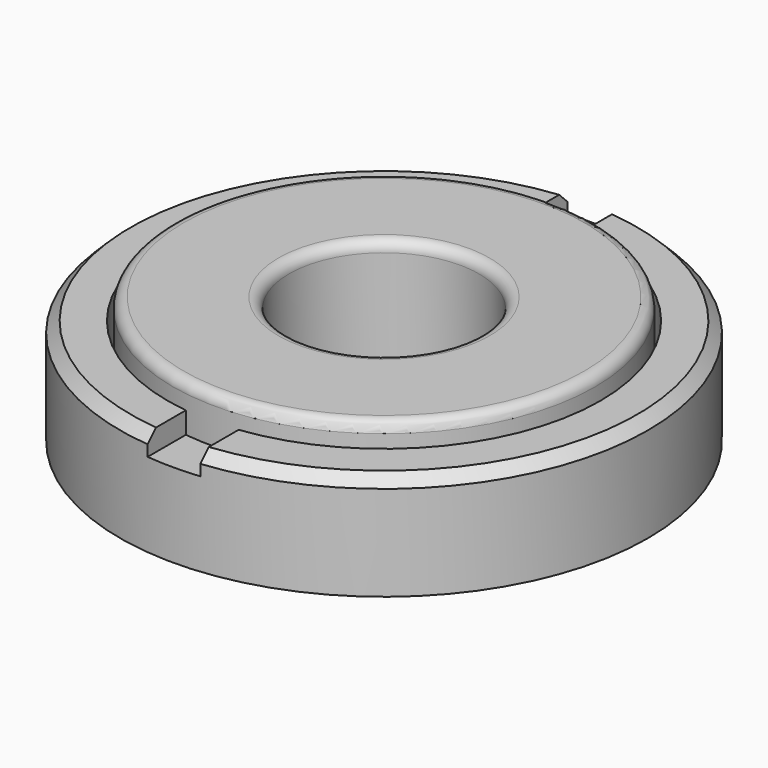
from build123d import *

# Parameters (mm, degrees)
F0_R     = 4
F1_DEPTH = 2.4
F0_R_2   = 5
F0_R_3   = 4.1
F2_DEPTH = 2
F3_D     = 3.6
F4_R     = 0.2
F5_SIZE  = 0.2
F6_W     = 1
F6_H     = 0.5
F7_DEPTH = 25


with BuildPart() as f1:
    # F0 (on Top) → F1 (new body)
    with BuildSketch(Plane.XY):
        Circle(F0_R)
    extrude(amount=F1_DEPTH)

    # F3 (through all)
    with Locations(Plane(origin=(0, 0, 0), x_dir=(1, 0, 0), z_dir=(0, 0, -1))):
        with Locations((0, 0)):
            Hole(F3_D / 2)

    # F4
    f4_edges = [f1.edges().sort_by_distance(p)[0] for p in [
        (-4, 0, 2.4),
        (-1.8, 0, 2.4),
    ]]
    fillet(f4_edges, radius=F4_R)


with BuildPart() as f2:
    # F0 (on Top) → F2 (new body)
    with BuildSketch(Plane.XY):
        Circle(F0_R_2)
        Circle(F0_R_3, mode=Mode.SUBTRACT)
    extrude(amount=F2_DEPTH)

    # F5
    f5_edges = [f2.edges().sort_by_distance(p)[0] for p in [
        (-5, 0, 2),
    ]]
    chamfer(f5_edges, length=F5_SIZE)


with BuildPart() as f7:
    # F6 (on Front) → F7 (new body)
    with BuildSketch(Plane.XZ):
        with Locations((0.5, 1.8409643844)):
            Rectangle(F6_W, F6_H)
    extrude(amount=F7_DEPTH)


with BuildPart() as f7_1:
    # F8: moved
    add(f7.part.moved(Location((-0.5, 13.3, 0))))


with BuildPart() as f2_1:
    add(f2.part)

    # F9: cut F7
    add(f7_1.part, mode=Mode.SUBTRACT)


solid = Compound([f1.part, f2_1.part])
